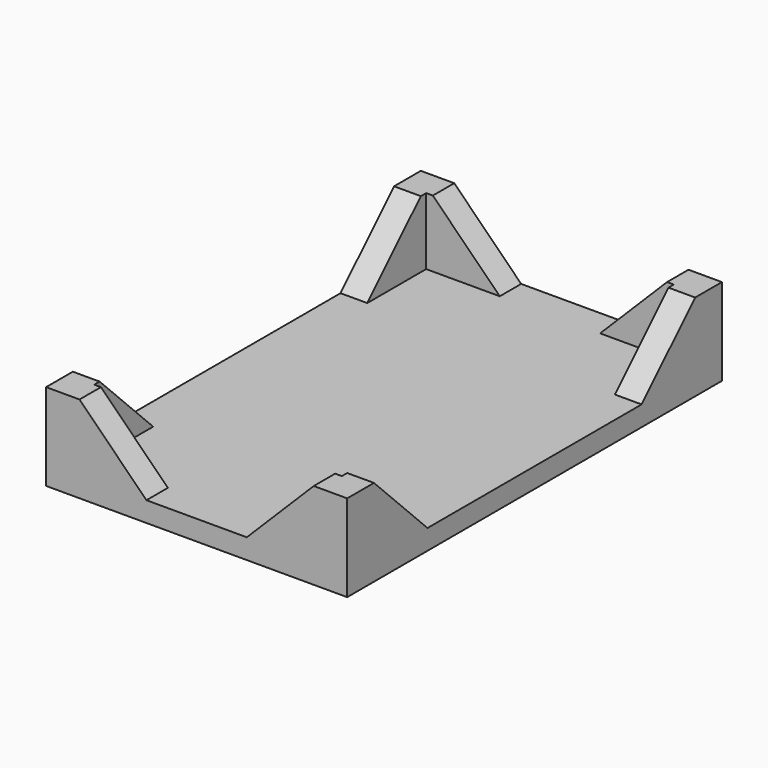
from build123d import *

# Parameters (mm, degrees)
F0_W     = 45
F0_H     = 70
F1_DEPTH = 3
F3_DEPTH = 10
F4_SIZE  = 9.99999


# Not quite as in the source:
# - a fillet or chamfer is up to 0.001 mm smaller than in the source, because OpenCascade refuses the exact size


with BuildPart() as f1:
    # F0 (on Top) → F1 (new body)
    with BuildSketch(Plane.XY):
        Rectangle(F0_W, F0_H)
    extrude(amount=F1_DEPTH)

    # F2 (on face) → F3 (join)
    with BuildSketch(Plane.XY.offset(3)):
        Polygon((-18.5, 20), (-18.5, 31), (-7.5, 31), (-7.5, 35), (-22.5, 35), (-22.5, 20), align=None)
        Polygon((7.5, 35), (7.5, 31), (18.5, 31), (18.5, 20), (22.5, 20), (22.5, 35), align=None)
        Polygon((18.5, -31), (7.5, -31), (7.5, -35), (22.5, -35), (22.5, -20), (18.5, -20), align=None)
        Polygon((-18.5, -31), (-18.5, -20), (-22.5, -20), (-22.5, -35), (-7.5, -35), (-7.5, -31), align=None)
    extrude(amount=F3_DEPTH)

    # F4 (size 10 in the source; OpenCascade refuses exactly that, so slightly less here)
    f4_edges = [f1.edges().sort_by_distance(p)[0] for p in [
        (-7.5, 33, 13),
        (-7.5, -33, 13),
        (-20.5, -20, 13),
        (20.5, -20, 13),
        (20.5, 20, 13),
        (-20.5, 20, 13),
        (7.5, -33, 13),
        (7.5, 33, 13),
    ]]
    chamfer(f4_edges, length=F4_SIZE)


solid = f1.part
